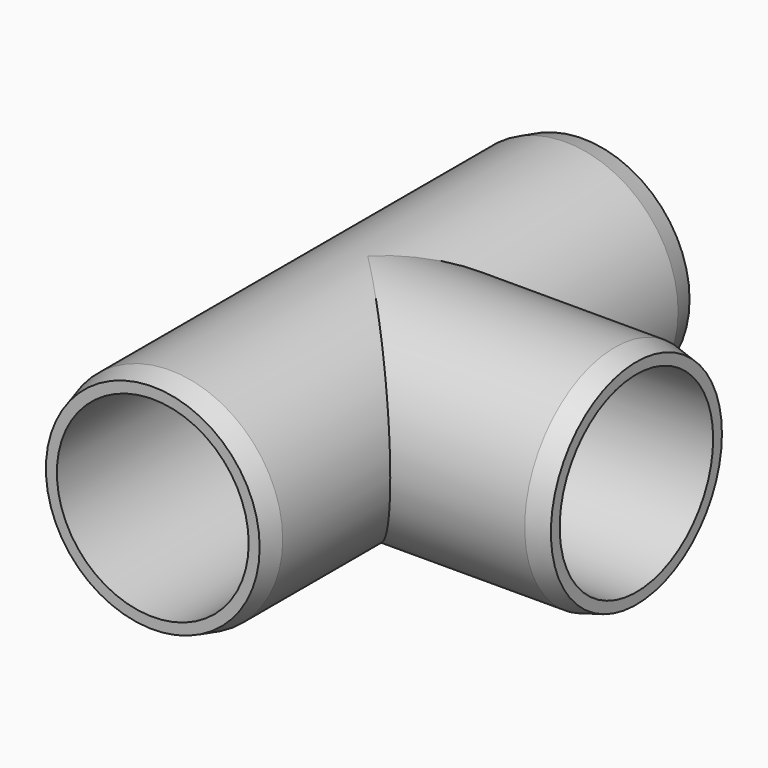
from build123d import *

# Parameters (mm, degrees)
F0_R          = 24.765
F0_R_2        = 21.082
F1_DEPTH      = 59.055
F2_R          = 24.765
F2_R_2        = 21.082
F3_DEPTH      = 59.055
F4_DEPTH      = 59.0560001
F5_DEPTH      = 59.0560001
F5_DEPTH_BACK = 59.0560001
F6_SIZE2      = 1.27
F6_SIZE       = 4.7397045256
F6_2_SIZE2    = 1.27
F6_2_SIZE     = 4.7397045256


# Not quite as in the source:
# - two fillets or chamfers of one size are made in one step


with BuildPart() as f1:
    # F0 (on Front) → F1 (new body, symmetric)
    with BuildSketch(Plane.XZ):
        Circle(F0_R)
        Circle(F0_R_2, mode=Mode.SUBTRACT)
    extrude(amount=F1_DEPTH, both=True)

    # F2 (on Right) → F3 (join)
    with BuildSketch(Plane.YZ):
        Circle(F2_R)
        Circle(F2_R_2, mode=Mode.SUBTRACT)
    extrude(amount=F3_DEPTH)

    # F2 (on Right) → F4 (cut, through all)
    with BuildSketch(Plane.YZ):
        Circle(F2_R_2)
    extrude(amount=F4_DEPTH, mode=Mode.SUBTRACT)

    # F0 (on Front) → F5 (cut, two sides)
    with BuildSketch(Plane.XZ) as f5_sk:
        Circle(F0_R_2)
    extrude(amount=F5_DEPTH, mode=Mode.SUBTRACT)
    extrude(f5_sk.sketch, amount=-F5_DEPTH_BACK, mode=Mode.SUBTRACT)

    # F6
    f6_edges = [f1.edges().sort_by_distance(p)[0] for p in [
        (-24.765, -59.055, 0),
        (-24.765, 59.055, 0),
    ]]
    f6_side = f1.faces().sort_by_distance((-24.765, 0, 0))[0]
    chamfer(f6_edges, length=F6_SIZE, length2=F6_SIZE2, reference=f6_side)

    # F6#2
    f6_2_edges = [f1.edges().sort_by_distance(p)[0] for p in [
        (59.055, -24.765, 0),
    ]]
    f6_2_side = f1.faces().sort_by_distance((29.5275, -24.765, 0))[0]
    chamfer(f6_2_edges, length=F6_2_SIZE, length2=F6_2_SIZE2, reference=f6_2_side)


solid = f1.part
